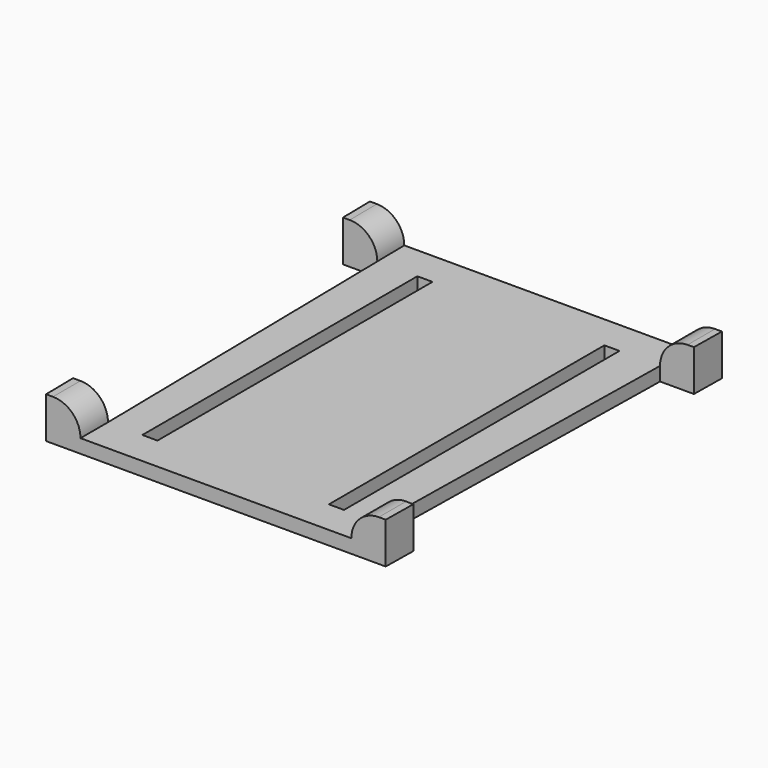
from build123d import *

# Parameters (mm, degrees)
F0_W     = 25
F0_H     = 50
F1_DEPTH = 2
F2_DEPTH = 6
F3_R     = 3.99999


# Not quite as in the source:
# - a fillet or chamfer is up to 0.001 mm smaller than in the source, because OpenCascade refuses the exact size


with BuildPart() as f1:
    # F0 (on Top) → F1 (new body)
    with BuildSketch(Plane.XY):
        Polygon((8.9700092217, 2.9870720308), (8.9700092217, -2.0129279692), (48.3700092217, -2.0129279692), (48.3700092217, 2.9870720308), (49.2700092217, 52.9870720308), (49.2700092217, 57.9870720308), (8.0700092217, 57.9870720308), (8.1450092217, 52.9870720308), align=None)
        Polygon((41.1700092217, 2.9040758964), (41.1700092217, 2.9870720308), (16.1700092217, 2.9870720308), (13.9700092217, 2.9870720308), (13.9700092217, 52.9870720308), (16.1700092217, 52.9870720308), (41.1700092217, 52.9870720308), (43.3700092217, 52.9870720308), (43.3700092217, 2.9040758964), align=None, mode=Mode.SUBTRACT)
        Polygon((49.2700092217, 57.9870720308), (49.2700092217, 52.9870720308), (54.1950092217, 52.9870720308), (54.2700092217, 57.9870720308), align=None)
        Polygon((3.0700092217, 57.9870720308), (3.1450092217, 52.9870720308), (8.1450092217, 52.9870720308), (8.0700092217, 57.9870720308), align=None)
        Polygon((3.8950092217, 2.9870720308), (3.9700092217, -2.0129279692), (8.9700092217, -2.0129279692), (8.9700092217, 2.9870720308), align=None)
        Polygon((48.3700092217, 2.9870720308), (48.3700092217, -2.0129279692), (53.3700092217, -2.0129279692), (53.4438676036, 2.910964155), align=None)
        with Locations((28.6700092217, 27.9870720308)):
            Rectangle(F0_W, F0_H)
    extrude(amount=F1_DEPTH)

    # F0 (on Top) → F2 (join)
    with BuildSketch(Plane.XY):
        Polygon((3.8950092217, 2.9870720308), (3.9700092217, -2.0129279692), (8.9700092217, -2.0129279692), (8.9700092217, 2.9870720308), align=None)
        Polygon((48.3700092217, 2.9870720308), (48.3700092217, -2.0129279692), (53.3700092217, -2.0129279692), (53.4438676036, 2.910964155), align=None)
        Polygon((49.2700092217, 57.9870720308), (49.2700092217, 52.9870720308), (54.1950092217, 52.9870720308), (54.2700092217, 57.9870720308), align=None)
        Polygon((3.0700092217, 57.9870720308), (3.1450092217, 52.9870720308), (8.1450092217, 52.9870720308), (8.0700092217, 57.9870720308), align=None)
    extrude(amount=F2_DEPTH)

    # F3 (radius 4 in the source; OpenCascade refuses exactly that, so slightly less here)
    f3_edges = [f1.edges().sort_by_distance(p)[0] for p in [
        (8.970009, 0.487072, 6),
        (8.107509, 55.487072, 6),
        (49.270009, 55.487072, 6),
        (48.370009, 0.487072, 6),
    ]]
    fillet(f3_edges, radius=F3_R)


solid = f1.part
